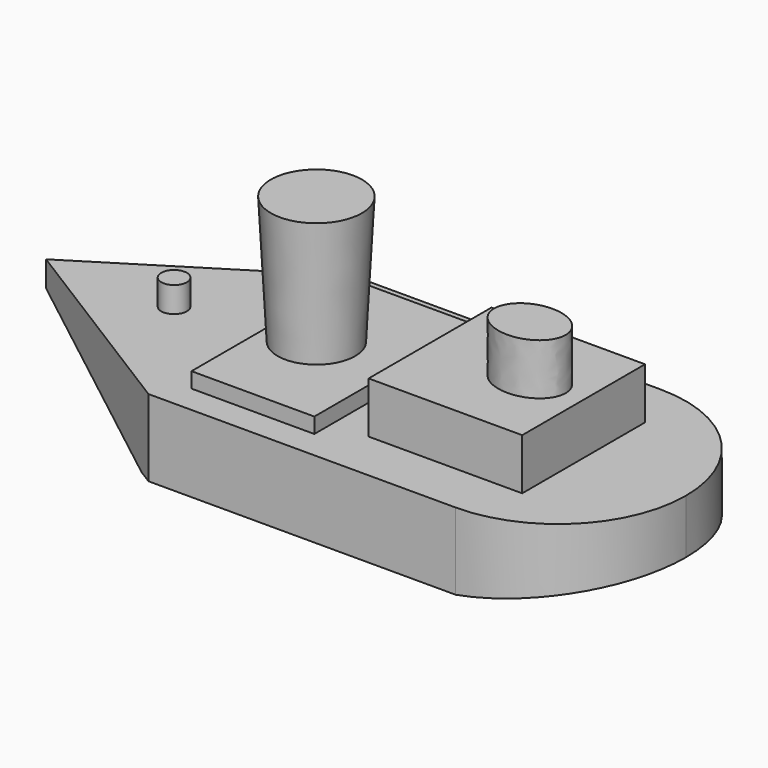
from build123d import *

# Parameters (mm, degrees)
F0_W      = 125
F0_H      = 15
F1_DEPTH  = 25
F2_R      = 24.99999
F4_DEPTH  = 50.001
F6_DEPTH  = 25
F8_DEPTH  = 50.001
F9_W      = 30
F9_H      = 30
F10_DEPTH = 10
F11_W     = 20
F11_H     = 5
F12_DEPTH = 17.5
F14_DEPTH = 10
F15_R     = 2.5
F16_DEPTH = 5
F21_DEPTH = 25
F18_W     = 24
F18_H     = 39
F18_W_2   = 20
F18_H_2   = 35
F19_DEPTH = 3
F20_R     = 7.5835339327
F22_DEPTH = 25
F22_TAPER = -3


# Not quite as in the source:
# - a fillet or chamfer is up to 0.001 mm smaller than in the source, because OpenCascade refuses the exact size


with BuildPart() as f1:
    # F0 (on Front) → F1 (new body, symmetric)
    with BuildSketch(Plane.XZ):
        Rectangle(F0_W, F0_H)
    extrude(amount=F1_DEPTH, both=True)

    # F2 (radius 25 in the source; OpenCascade refuses exactly that, so slightly less here)
    f2_edges = [f1.edges().sort_by_distance(p)[0] for p in [
        (62.5, -25, 0),
        (62.5, 25, 0),
    ]]
    fillet(f2_edges, radius=F2_R)

    # F3 (on face) → F4 (cut, through all)
    with BuildSketch(Plane.XZ.offset(25)):
        Polygon((-25.1794919243, -7.5), (-62.5, 2.5), (-62.5, -7.5), align=None)
    extrude(amount=-F4_DEPTH, mode=Mode.SUBTRACT)

    # F5 (on face) → F6 (cut)
    with BuildSketch(Plane.XY.offset(7.5)):
        Polygon((-22.5, -25), (-62.5, 0), (-62.5, -25), align=None)
        Polygon((-62.5, 25), (-62.5, 0), (-22.5, 25), align=None)
    extrude(amount=-F6_DEPTH, mode=Mode.SUBTRACT)

    # F7 (on face) → F8 (cut, through all)
    with BuildSketch(Plane.XZ.offset(25)):
        Polygon((96.8128483375, 2.9584554646), (37.5, -7.5), (96.8128483375, -7.5), align=None)
    extrude(amount=-F8_DEPTH, mode=Mode.SUBTRACT)

    # F11 (on Front) → F12 (cut, symmetric)
    with BuildSketch(Plane.XZ):
        with Locations((-6.5, 5)):
            Rectangle(F11_W, F11_H)
    extrude(amount=F12_DEPTH, both=True, mode=Mode.SUBTRACT)


with BuildPart() as f10:
    # F9 (on face) → F10 (new body)
    with BuildSketch(Plane.XY.offset(7.5)):
        with Locations((27.5, 0)):
            Rectangle(F9_W, F9_H)
    extrude(amount=F10_DEPTH)


with BuildPart() as f14:
    # F13 (on face) → F14 (new body)
    with BuildSketch(Plane.XY.offset(17.5)):
        with BuildLine():
            add(Edge.make_bspline(
                [(25, 0), (25, -9.5262794416), (35.5, -4.7631397208), (46, 0), (35.5, 4.7631397208), (25, 9.5262794416), (25, 0)],
                knots=[0, 0, 0, 2.0943951024, 2.0943951024, 4.1887902048, 4.1887902048, 6.2831853072, 6.2831853072, 6.2831853072], degree=2, weights=[1, 0.5, 1, 0.5, 1, 0.5, 1]))
        make_face()
    extrude(amount=F14_DEPTH)


with BuildPart() as f16:
    # F15 (on face) → F16 (new body)
    with BuildSketch(Plane.XY.offset(7.5)):
        with Locations((-37.5, 0)):
            Circle(F15_R)
    extrude(amount=F16_DEPTH)


with BuildPart() as f21:
    # F21 (new): a face of the model
    f21_faces = [f1.part.faces().sort_by_distance(p)[0] for p in [
        (8.9797168321, 0, 7.5),
    ]]
    extrude(f21_faces, amount=F21_DEPTH)


with BuildPart() as f19:
    # F18 (on face) → F19 (new body)
    with BuildSketch(Plane.XY.offset(7.5)):
        with Locations((-6.5, 0)):
            Rectangle(F18_W, F18_H)
        with Locations((-6.5, 0)):
            Rectangle(F18_W_2, F18_H_2, mode=Mode.SUBTRACT)
        with Locations((-6.5, 0)):
            Rectangle(F18_W_2, F18_H_2)
    extrude(amount=F19_DEPTH)

    # F20 (on face) → F22 (join)
    with BuildSketch(Plane.XY.offset(10.5)):
        with Locations((-9.6975341439, 0)):
            Circle(F20_R)
    extrude(amount=F22_DEPTH, taper=F22_TAPER)


solid = Compound([f1.part, f10.part, f14.part, f16.part, f19.part])
